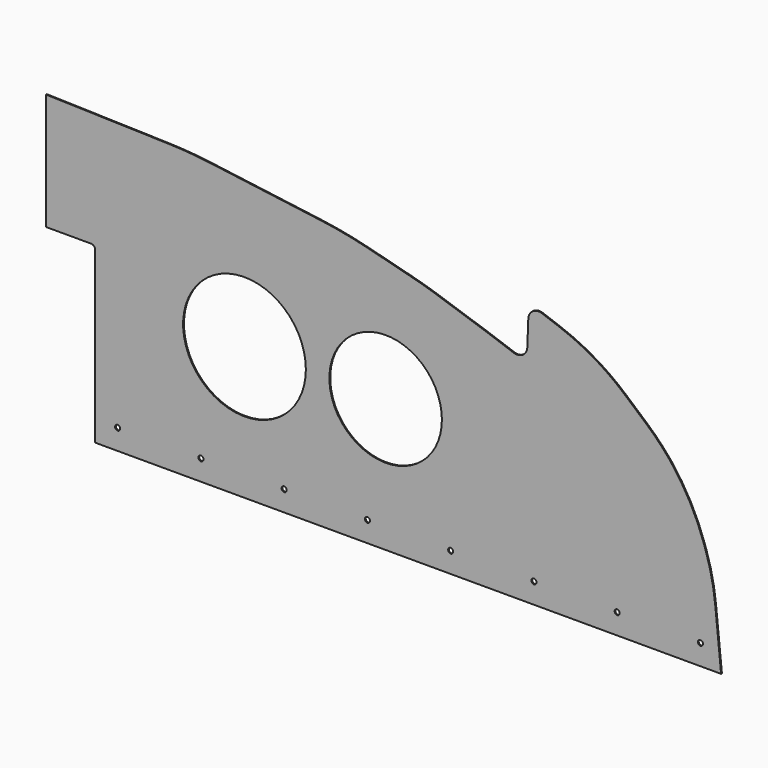
from build123d import *

# Parameters (mm, degrees)
F0_R        = 1.25
F0_R_2      = 30
F0_R_3      = 27.5
F1_DEPTH    = 0.5
F2_R        = 2
F3_R        = 5
F4_R        = 200
F5_T1_DEPTH = 35.8886959127
F6_T1_DEPTH = 56.2497974387
F6_T3_DEPTH = 89.6754808083
F6_T5_DEPTH = 45.7004795966
F6_T7_DEPTH = 39.8671139621
F6_T9_DEPTH = 53.963301214


# Not quite as in the source:
# - a fillet or chamfer that OpenCascade refuses, or shapes differently, is made with other operations: its cross-section is extruded or revolved along the edge and cut away or added


with BuildPart() as f1:
    # F0 (on Front) → F1 (new body)
    with BuildSketch(Plane.XZ):
        Polygon((24, 85), (24, 0), (330, 0), (326, 40), (316, 70), (300, 90), (277, 110), (261, 120), (236, 129), (235, 103), (215, 110), (185, 120), (146, 130), (70, 140), (0, 142), (0, 85), align=None)
        with Locations((35, 10)):
            Circle(F0_R, mode=Mode.SUBTRACT)
        with Locations((75.7, 10)):
            Circle(F0_R, mode=Mode.SUBTRACT)
        with Locations((116.4, 10)):
            Circle(F0_R, mode=Mode.SUBTRACT)
        with Locations((157.1, 10)):
            Circle(F0_R, mode=Mode.SUBTRACT)
        with Locations((97, 65)):
            Circle(F0_R_2, mode=Mode.SUBTRACT)
        with Locations((197.8, 10)):
            Circle(F0_R, mode=Mode.SUBTRACT)
        with Locations((238.5, 10)):
            Circle(F0_R, mode=Mode.SUBTRACT)
        with Locations((279.2, 10)):
            Circle(F0_R, mode=Mode.SUBTRACT)
        with Locations((319.9, 10)):
            Circle(F0_R, mode=Mode.SUBTRACT)
        with Locations((166, 65)):
            Circle(F0_R_3, mode=Mode.SUBTRACT)
    extrude(amount=F1_DEPTH)

    # F2
    f2_edges = [f1.edges().sort_by_distance(p)[0] for p in [
        (24, -0.25, 85),
    ]]
    fillet(f2_edges, radius=F2_R)

    # F3
    f3_edges = [f1.edges().sort_by_distance(p)[0] for p in [
        (235, -0.25, 103),
        (236, -0.25, 129),
    ]]
    fillet(f3_edges, radius=F3_R)

    # F4
    f4_edges = [f1.edges().sort_by_distance(p)[0] for p in [
        (70, -0.25, 140),
        (146, -0.25, 130),
    ]]
    fillet(f4_edges, radius=F4_R)

    # F5: fillet of radius 200 on 1 edges, made by hand

    # F5_s2 → F5_t1 (cut)
    with BuildSketch(Plane.XZ.offset(-17.6943479563)):
        with BuildLine():
            ThreePointArc((178.1440498006, 121.7579359486), (184.9646346256, 119.8799020084), (191.7145329504, 117.7618223499))
            Line((191.7145329504, 117.7618223499), (185, 120))
            Line((185, 120), (178.1440498006, 121.7579359486))
        make_face()
    extrude(amount=F5_T1_DEPTH, mode=Mode.SUBTRACT)

    # F6: fillet of radius 100 on 5 edges, made by hand

    # F6_s2 → F6_t1 (cut)
    with BuildSketch(Plane.XZ.offset(-27.8748987193)):
        with BuildLine():
            ThreePointArc((322.47407322, 50.57778034), (325.3940178786, 39.8703898792), (327.109462436, 28.9053756404))
            Line((327.109462436, 28.9053756404), (326, 40))
            Line((326, 40), (322.47407322, 50.57778034))
        make_face()
    extrude(amount=F6_T1_DEPTH, mode=Mode.SUBTRACT)

    # F6_s4 → F6_t3 (cut)
    with BuildSketch(Plane.XZ.offset(-44.5877404042)):
        with BuildLine():
            ThreePointArc((304.8585037552, 83.9268703061), (314.6138472293, 69.2458956516), (321.6399526159, 53.0801421523))
            Line((321.6399526159, 53.0801421523), (316, 70))
            Line((316, 70), (304.8585037552, 83.9268703061))
        make_face()
    extrude(amount=F6_T3_DEPTH, mode=Mode.SUBTRACT)

    # F6_s6 → F6_t5 (cut)
    with BuildSketch(Plane.XZ.offset(-22.6002397983)):
        with BuildLine():
            ThreePointArc((293.1782936984, 95.9319185231), (299.7058017999, 89.7176239908), (305.6473031502, 82.9408710622))
            Line((305.6473031502, 82.9408710622), (300, 90))
            Line((300, 90), (293.1782936984, 95.9319185231))
        make_face()
    extrude(amount=F6_T5_DEPTH, mode=Mode.SUBTRACT)

    # F6_s8 → F6_t7 (cut)
    with BuildSketch(Plane.XZ.offset(-19.683556981)):
        with BuildLine():
            ThreePointArc((270.3233508253, 114.1729057342), (276.8158857708, 109.7512495983), (282.9413283175, 104.83362755))
            Line((282.9413283175, 104.83362755), (277, 110))
            Line((277, 110), (270.3233508253, 114.1729057342))
        make_face()
    extrude(amount=F6_T7_DEPTH, mode=Mode.SUBTRACT)

    # F6_s10 → F6_t9 (cut)
    with BuildSketch(Plane.XZ.offset(-26.731650607)):
        with BuildLine():
            ThreePointArc((250.9394105782, 123.6218121919), (260.7509863663, 119.487225172), (270.0673577512, 114.3329014055))
            Line((270.0673577512, 114.3329014055), (261, 120))
            Line((261, 120), (250.9394105782, 123.6218121919))
        make_face()
    extrude(amount=F6_T9_DEPTH, mode=Mode.SUBTRACT)


solid = f1.part
